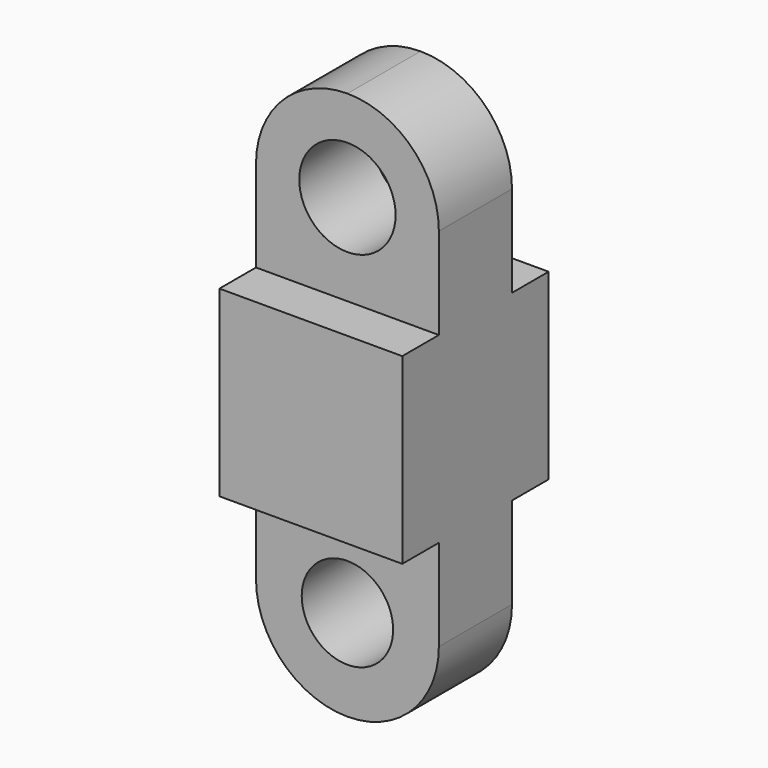
from build123d import *

# Parameters (mm, degrees)
F0_W     = 40
F0_H     = 120
F1_DEPTH = 10
F2_W     = 40
F2_H     = 40
F3_DEPTH = 10
F5_R     = 10.5368442401
F6_DEPTH = 20
F7_R     = 10
F8_DEPTH = 20
F9_R     = 19.99999
F10_R    = 19.99999


# Not quite as in the source:
# - a fillet or chamfer is up to 0.001 mm smaller than in the source, because OpenCascade refuses the exact size


with BuildPart() as f1:
    # F0 (on Front) → F1 (new body)
    with BuildSketch(Plane.XZ):
        Rectangle(F0_W, F0_H)
    extrude(amount=F1_DEPTH)

    # F2 (on face) → F3 (join)
    with BuildSketch(Plane.XZ.offset(10)):
        Rectangle(F2_W, F2_H)
    extrude(amount=F3_DEPTH)

    # F4: F1 across face


with BuildPart() as f1_1:
    add(f1.part)
    add(f1.part.mirror(Plane(origin=(0, 0, 0), x_dir=(1, 0, 0), z_dir=(0, 1, 0))))

    # F5 (on face) → F6 (cut, through all)
    with BuildSketch(Plane.XZ.offset(10)):
        with Locations((0, 40)):
            Circle(F5_R)
    extrude(amount=-F6_DEPTH, mode=Mode.SUBTRACT)

    # F7 (on face) → F8 (cut, through all)
    with BuildSketch(Plane(origin=(0, 10, 0), x_dir=(-1, 0, 0), z_dir=(0, 1, 0))):
        with Locations((0, -40)):
            Circle(F7_R)
    extrude(amount=-F8_DEPTH, mode=Mode.SUBTRACT)

    # F9 (radius 20 in the source; OpenCascade refuses exactly that, so slightly less here)
    f9_edges = [f1_1.edges().sort_by_distance(p)[0] for p in [
        (-20, 0, 60),
        (20, 0, 60),
    ]]
    fillet(f9_edges, radius=F9_R)

    # F10 (radius 20 in the source; OpenCascade refuses exactly that, so slightly less here)
    f10_edges = [f1_1.edges().sort_by_distance(p)[0] for p in [
        (20, 0, -60),
        (-20, 0, -60),
    ]]
    fillet(f10_edges, radius=F10_R)


solid = f1_1.part
